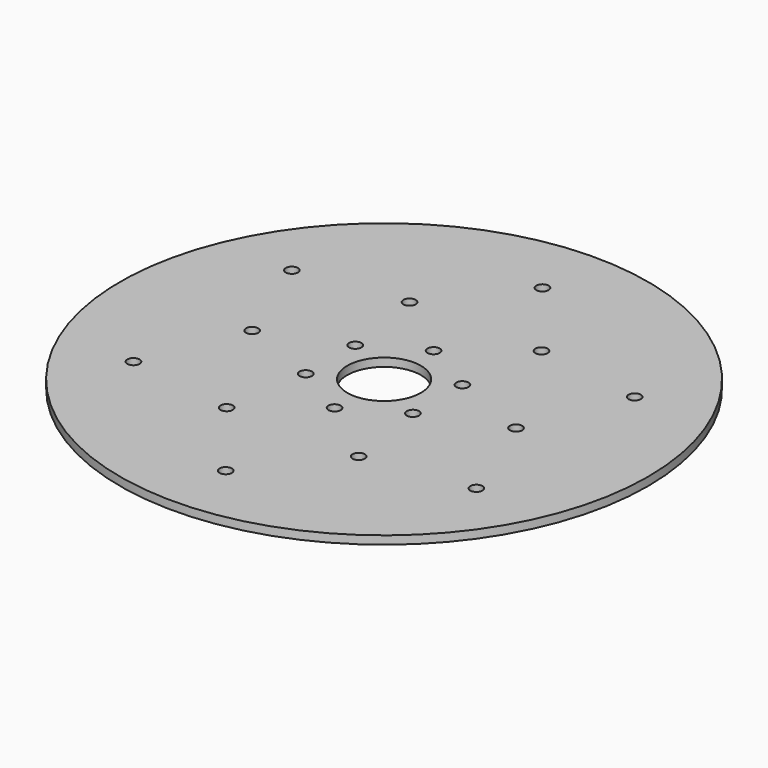
from build123d import *

# Parameters (mm, degrees)
F0_R            = 101.6
F0_R_2          = 14.1605
F1_DEPTH        = 3.175
F2_R            = 2.3622
F3_DEPTH        = 3.176
F3_COPIES_COUNT = 6


# Not quite as in the source:
# - a pattern or mirror of a feature is missing from the dataset's text; its kind, count and spacing are read off the source's solid


with BuildPart() as f1:
    # F0 (on Top) → F1 (new body)
    with BuildSketch(Plane.XY):
        Circle(F0_R)
        Circle(F0_R_2, mode=Mode.SUBTRACT)
    extrude(amount=F1_DEPTH)

    # F2 (on face) → F3 (cut, through all)
    with BuildSketch(Plane.XY.offset(3.175)):
        with Locations((0, 23.8125)):
            Circle(F2_R)
        with Locations((0, 76.2)):
            Circle(F2_R)
        with Locations((25.4, 43.9940905122)):
            Circle(F2_R)
    f3 = extrude(amount=-F3_DEPTH, mode=Mode.SUBTRACT)

    # F3_copies: F3 ×6 about axis
    f3_copies_axis = Axis((0, 0, 0), (0, 0, 1))
    for i in range(1, F3_COPIES_COUNT):
        add(f3.rotate(f3_copies_axis, i * 360 / F3_COPIES_COUNT), mode=Mode.SUBTRACT)


solid = f1.part
